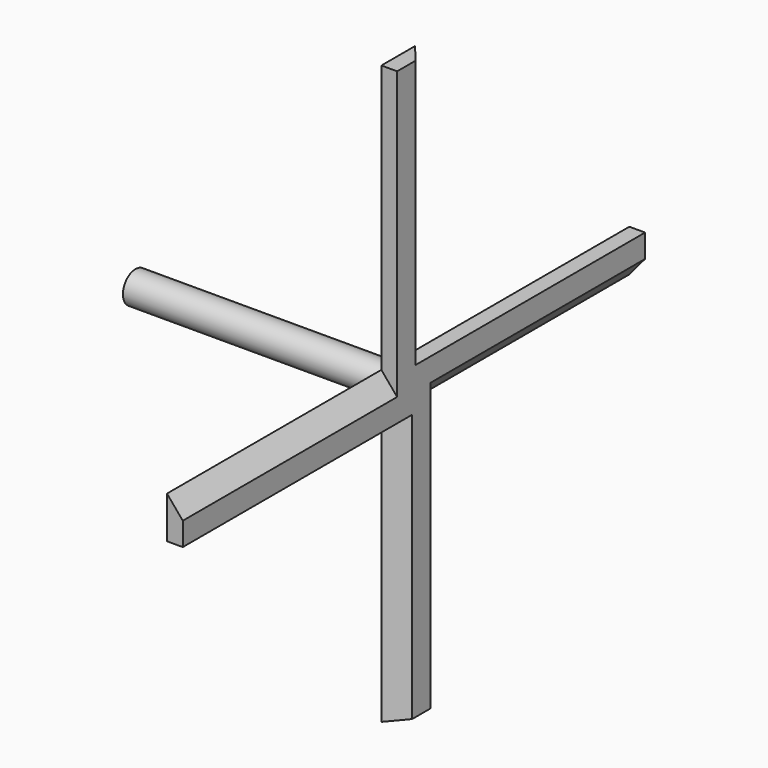
from build123d import *

# Parameters (mm, degrees)
F0_R          = 3.81
F1_DEPTH      = 12.7
F1_DEPTH_BACK = 50.8
F2_W          = 64.77
F2_H          = 10.16
F2_W_2        = 10.16
F2_H_2        = 64.77
F3_DEPTH      = 3.81
F4_SIZE2      = 4.540571
F4_SIZE       = 3.80999
F4_2_SIZE2    = 4.540571
F4_2_SIZE     = 3.80999
F4_3_SIZE2    = 4.540571
F4_3_SIZE     = 3.80999
F4_4_SIZE2    = 4.540571
F4_4_SIZE     = 3.80999


# Not quite as in the source:
# - a fillet or chamfer is up to 0.001 mm smaller than in the source, because OpenCascade refuses the exact size


with BuildPart() as f1:
    # F0 (on Right) → F1 (new body, two sides)
    with BuildSketch(Plane.YZ) as f1_sk:
        Circle(F0_R)
    extrude(amount=F1_DEPTH)
    extrude(f1_sk.sketch, amount=-F1_DEPTH_BACK)

    # F2 (on face) → F3 (join)
    with BuildSketch(Plane.YZ.offset(12.7)):
        with Locations((37.465, 0)):
            Rectangle(F2_W, F2_H)
        Rectangle(F2_W_2, F2_H)
        with Locations((0, 37.465)):
            Rectangle(F2_W_2, F2_H_2)
        with Locations((-37.465, 0)):
            Rectangle(F2_W, F2_H)
        with Locations((0, -37.465)):
            Rectangle(F2_W_2, F2_H_2)
    extrude(amount=F3_DEPTH)

    # F4 (size 3.81 and 4.5405811878 in the source; OpenCascade refuses exactly that, so slightly less here)
    f4_edges = [f1.edges().sort_by_distance(p)[0] for p in [
        (16.51, 5.08, 37.465),
    ]]
    f4_side = f1.faces().sort_by_distance((14.605, 5.08, 37.465))[0]
    chamfer(f4_edges, length=F4_SIZE, length2=F4_SIZE2, reference=f4_side)

    # F4#2 (size 3.81 and 4.5405811878 in the source; OpenCascade refuses exactly that, so slightly less here)
    f4_2_edges = [f1.edges().sort_by_distance(p)[0] for p in [
        (16.51, 37.465, -5.08),
    ]]
    f4_2_side = f1.faces().sort_by_distance((14.605, 37.465, -5.08))[0]
    chamfer(f4_2_edges, length=F4_2_SIZE, length2=F4_2_SIZE2, reference=f4_2_side)

    # F4#3 (size 3.81 and 4.5405811878 in the source; OpenCascade refuses exactly that, so slightly less here)
    f4_3_edges = [f1.edges().sort_by_distance(p)[0] for p in [
        (16.51, -5.08, -37.465),
    ]]
    f4_3_side = f1.faces().sort_by_distance((14.605, -5.08, -37.465))[0]
    chamfer(f4_3_edges, length=F4_3_SIZE, length2=F4_3_SIZE2, reference=f4_3_side)

    # F4#4 (size 3.81 and 4.5405811878 in the source; OpenCascade refuses exactly that, so slightly less here)
    f4_4_edges = [f1.edges().sort_by_distance(p)[0] for p in [
        (16.51, -37.465, 5.08),
    ]]
    f4_4_side = f1.faces().sort_by_distance((14.605, -37.465, 5.08))[0]
    chamfer(f4_4_edges, length=F4_4_SIZE, length2=F4_4_SIZE2, reference=f4_4_side)


solid = f1.part
